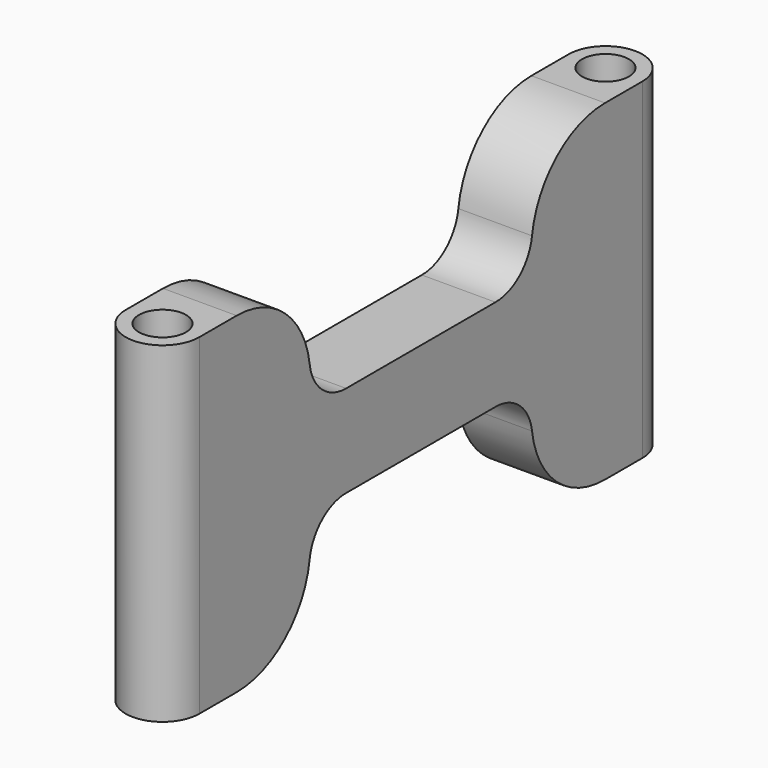
from build123d import *

# Parameters (mm, degrees)
F0_R     = 2.55
F1_DEPTH = 36
F2_W     = 30
F2_H     = 13
F3_DEPTH = 8
F4_R     = 10
F5_R     = 5


with BuildPart() as f1:
    # F0 (on Top) → F1 (new body)
    with BuildSketch(Plane.XY):
        with BuildLine():
            ThreePointArc((4, 30.065), (0, 34.065), (-4, 30.065))
            Line((-4, 30.065), (-4, -30.065))
            ThreePointArc((-4, -30.065), (0, -34.065), (4, -30.065))
            Line((4, -30.065), (4, 30.065))
        make_face()
        with Locations((0, -30.065)):
            Circle(F0_R, mode=Mode.SUBTRACT)
        with Locations((0, 30.065)):
            Circle(F0_R, mode=Mode.SUBTRACT)
    extrude(amount=F1_DEPTH)

    # F2 (on face) → F3 (cut, through all)
    with BuildSketch(Plane(origin=(-4, 0, 0), x_dir=(0, -1, 0), z_dir=(-1, 0, 0))):
        with Locations((0, 29.5)):
            Rectangle(F2_W, F2_H)
        with Locations((0, 6.5)):
            Rectangle(F2_W, F2_H)
    extrude(amount=-F3_DEPTH, mode=Mode.SUBTRACT)

    # F4
    f4_edges = [f1.edges().sort_by_distance(p)[0] for p in [
        (0, 15, 36),
        (0, 15, 0),
        (0, -15, 0),
        (0, -15, 36),
    ]]
    fillet(f4_edges, radius=F4_R)

    # F5
    f5_edges = [f1.edges().sort_by_distance(p)[0] for p in [
        (0, 15, 23),
        (0, -15, 23),
        (0, -15, 13),
        (0, 15, 13),
    ]]
    fillet(f5_edges, radius=F5_R)


solid = f1.part
